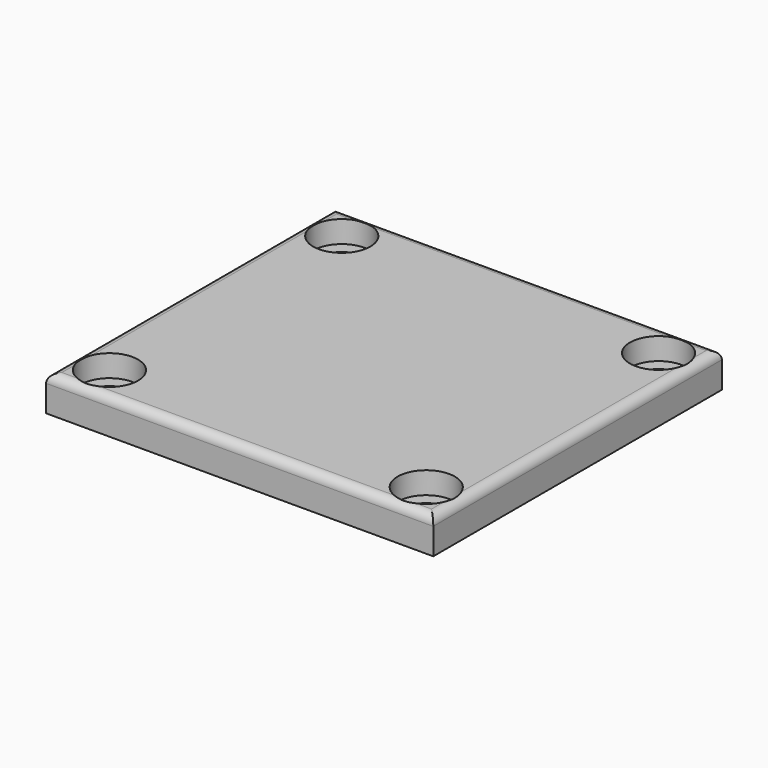
from build123d import *

# Parameters (mm, degrees)
F0_W        = 44
F0_H        = 41
F1_DEPTH    = 4
F2_R        = 1.75
F3_DEPTH    = 4.001
F4_R        = 3.25
F5_DEPTH    = 2.5
F6_T1_DEPTH = 46
F6_T3_DEPTH = 49


# Not quite as in the source:
# - a fillet or chamfer that OpenCascade refuses, or shapes differently, is made with other operations: its cross-section is extruded or revolved along the edge and cut away or added


with BuildPart() as f1:
    # F0 (on Top) → F1 (new body)
    with BuildSketch(Plane.XY):
        with Locations((17.9585738778, -18.5538536012)):
            Rectangle(F0_W, F0_H)
    extrude(amount=F1_DEPTH)

    # F2 (on face) → F3 (cut, through all)
    with BuildSketch(Plane.XY.offset(4)):
        with Locations((-0.0414261222, -2.0538536012)):
            Circle(F2_R)
        with Locations((35.9585738778, -2.0538536012)):
            Circle(F2_R)
        with Locations((35.9585738778, -35.0538536012)):
            Circle(F2_R)
        with Locations((-0.0414261222, -35.0538536012)):
            Circle(F2_R)
    extrude(amount=-F3_DEPTH, mode=Mode.SUBTRACT)

    # F4 (on face) → F5 (cut)
    with BuildSketch(Plane.XY.offset(4)):
        with Locations((-0.0414261222, -2.0538536012)):
            Circle(F4_R)
        with Locations((35.9585738778, -2.0538536012)):
            Circle(F4_R)
        with Locations((35.9585738778, -35.0538536012)):
            Circle(F4_R)
        with Locations((-0.0414261222, -35.0538536012)):
            Circle(F4_R)
    extrude(amount=-F5_DEPTH, mode=Mode.SUBTRACT)

    # F6: fillet of radius 1 on 4 edges, made by hand

    # F6_s2 → F6_t1 (cut)
    with BuildSketch(Plane.XZ.offset(-4.4461463988)):
        with BuildLine():
            ThreePointArc((-3.0414261222, 4), (-3.7485329034, 3.7071067812), (-4.0414261222, 3))
            Line((-4.0414261222, 3), (-4.0414261222, 4))
            Line((-4.0414261222, 4), (-3.0414261222, 4))
        make_face()
        with BuildLine():
            ThreePointArc((39.9585738778, 3), (39.665680659, 3.7071067812), (38.9585738778, 4))
            Line((38.9585738778, 4), (39.9585738778, 4))
            Line((39.9585738778, 4), (39.9585738778, 3))
        make_face()
    extrude(amount=F6_T1_DEPTH, mode=Mode.SUBTRACT)

    # F6_s4 → F6_t3 (cut)
    with BuildSketch(Plane.YZ.offset(-6.5414261222)):
        with BuildLine():
            ThreePointArc((-39.0538536012, 3), (-38.7609603824, 3.7071067812), (-38.0538536012, 4))
            Line((-38.0538536012, 4), (-39.0538536012, 4))
            Line((-39.0538536012, 4), (-39.0538536012, 3))
        make_face()
        with BuildLine():
            ThreePointArc((1.9461463988, 3), (1.65325318, 3.7071067812), (0.9461463988, 4))
            Line((0.9461463988, 4), (1.9461463988, 4))
            Line((1.9461463988, 4), (1.9461463988, 3))
        make_face()
    extrude(amount=F6_T3_DEPTH, mode=Mode.SUBTRACT)


solid = f1.part
